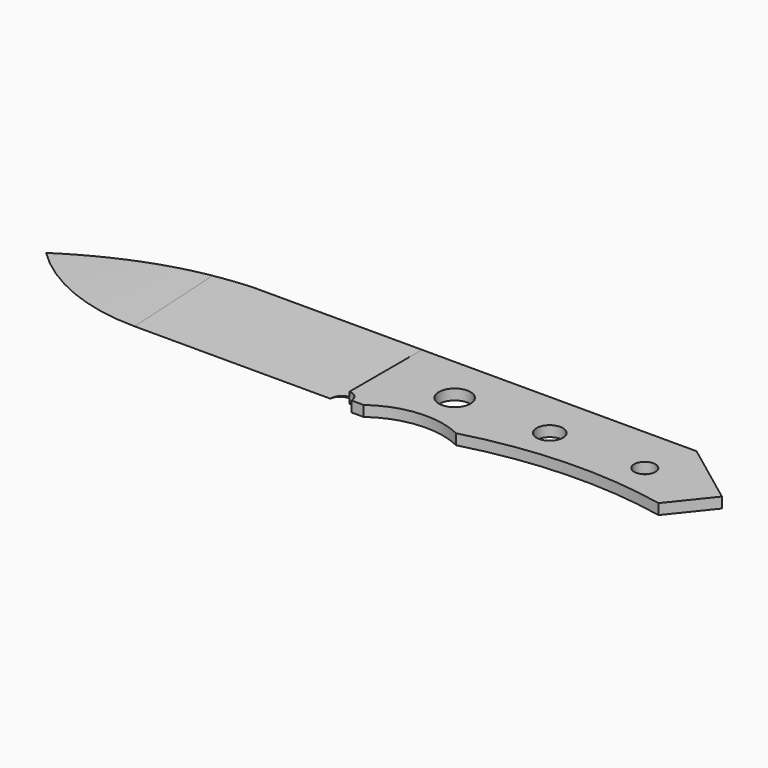
from build123d import *

# Parameters (mm, degrees)
F0_W     = 203.2
F0_H     = 38.1
F1_DEPTH = 3.175
F2_W     = 3.175
F2_H     = 4.445
F3_DEPTH = 25.4


# Not quite as in the source:
# - a feature names something its author has since deleted; it is built from what else it names


with BuildPart() as f1:
    # F0 (on Top) → F1 (new body)
    with BuildSketch(Plane.XY):
        with Locations((101.6, -19.05)):
            Rectangle(F0_W, F0_H)
    extrude(amount=F1_DEPTH)

    # F2 (on face) → F3 (cut)
    with BuildSketch(Plane.XY.offset(3.175)):
        with BuildLine():
            Line((0, -9.525), (0, -14.2875))
            ThreePointArc((0, -14.2875), (24.649723028, -4.4760985439), (50.8, 0))
            Line((50.8, 0), (0, 0))
            Line((0, 0), (0, -9.525))
        make_face()
        with Locations((103.1875, -35.8775)):
            Rectangle(F2_W, F2_H)
        with BuildLine():
            ThreePointArc((104.775, -30.48), (103.8450640303, -32.7250640303), (101.6, -33.655))
            Line((101.6, -33.655), (104.775, -33.655))
            Line((104.775, -33.655), (104.775, -30.48))
        make_face()
        with BuildLine():
            Line((104.775, -30.48), (101.6, -30.48))
            Line((101.6, -30.48), (101.6, -33.655))
            ThreePointArc((101.6, -33.655), (103.8450640303, -32.7250640303), (104.775, -30.48))
        make_face()
        with BuildLine():
            Line((101.6, -27.305), (101.6, -30.48))
            Line((101.6, -30.48), (104.775, -30.48))
            ThreePointArc((104.775, -30.48), (103.8450640303, -28.2349359697), (101.6, -27.305))
        make_face()
        with BuildLine():
            Line((98.4250000029, -30.4801362911), (101.6, -30.48))
            Line((101.6, -30.48), (101.6, -27.305))
            ThreePointArc((101.6, -27.305), (99.3548877841, -28.2349841564), (98.4250000029, -30.4801362911))
        make_face()
        with BuildLine():
            Line((101.6, -33.655), (101.6, -30.48))
            Line((101.6, -30.48), (98.4250000029, -30.4801362911))
            ThreePointArc((98.4250000029, -30.4801362911), (99.3549841564, -32.7251122159), (101.6, -33.655))
        make_face()
        with BuildLine():
            ThreePointArc((108.3690122037, -30.48), (106.4969075417, -31.9824905065), (104.775, -33.655))
            Line((104.775, -33.655), (104.775, -38.1))
            Line((104.775, -38.1), (184.15, -38.1))
            Line((184.15, -38.1), (193.675, -26.19375))
            ThreePointArc((193.675, -26.19375), (163.9135585822, -23.6655567526), (134.3847364187, -28.1581971794))
            ThreePointArc((134.3847364187, -28.1581971794), (121.0555708247, -25.7189035938), (108.3690122037, -30.48))
        make_face()
        with BuildLine():
            Line((101.6, -38.1), (101.6, -33.655))
            ThreePointArc((101.6, -33.655), (99.3549841564, -32.7251122159), (98.4250000029, -30.4801362911))
            Line((98.4250000029, -30.4801362911), (39.6036359929, -30.4826612755))
            ThreePointArc((39.6036359929, -30.4826612755), (18.2099329026, -26.2778753266), (0, -14.2875))
            Line((0, -14.2875), (0, -19.05))
            Line((0, -19.05), (0, -38.1))
            Line((0, -38.1), (101.6, -38.1))
        make_face()
        Polygon((203.2, 0), (184.15, 0), (203.2, -14.2875), align=None)
        Polygon((193.675, -26.19375), (184.15, -38.1), (203.2, -38.1), (203.2, -19.05), (203.2, -14.2875), align=None)
        with BuildLine():
            Line((108.3690122037, -30.48), (104.775, -30.48))
            Line((104.775, -30.48), (104.775, -33.655))
            ThreePointArc((104.775, -33.655), (106.4969075417, -31.9824905065), (108.3690122037, -30.48))
        make_face()
        with BuildLine():
            ThreePointArc((127.6218066335, -14.2875), (122.8593066335, -9.525), (118.0968066335, -14.2875))
            Line((118.0968066335, -14.2875), (127.6218066335, -14.2875))
        make_face()
        with BuildLine():
            Line((127.6218066335, -14.2875), (118.0968066335, -14.2875))
            ThreePointArc((118.0968066335, -14.2875), (122.8593066335, -19.05), (127.6218066335, -14.2875))
        make_face()
        with BuildLine():
            Line((176.8343066335, -14.2875), (183.1843066335, -14.2875))
            ThreePointArc((183.1843066335, -14.2875), (180.0093066335, -11.1125), (176.8343066335, -14.2875))
        make_face()
        with BuildLine():
            ThreePointArc((176.8343066335, -14.2875), (180.0093066335, -17.4625), (183.1843066335, -14.2875))
            Line((183.1843066335, -14.2875), (176.8343066335, -14.2875))
        make_face()
        with BuildLine():
            ThreePointArc((155.4030566335, -14.2875), (151.4343066335, -10.31875), (147.4655566335, -14.2875))
            Line((147.4655566335, -14.2875), (155.4030566335, -14.2875))
        make_face()
        with BuildLine():
            Line((155.4030566335, -14.2875), (147.4655566335, -14.2875))
            ThreePointArc((147.4655566335, -14.2875), (151.4343066335, -18.25625), (155.4030566335, -14.2875))
        make_face()
    extrude(amount=-F3_DEPTH, mode=Mode.SUBTRACT)

    # F8: sweep along a path in F5
    with BuildLine(Plane.XY.offset(1.5875)) as f8_path:
        Line((101.6, -30.48), (39.6036359929, -30.4826612755))
        ThreePointArc((39.6036359929, -30.4826612755), (18.2099329026, -26.2778753266), (0, -14.2875))
    # F7 (on offset) → F8 (sweep, cut)
    with BuildSketch(Plane.YZ.offset(101.6)):
        Polygon((-30.48, 3.1877), (-30.48, 1.5875), (-21.4048148322, 3.1877), align=None)
        Polygon((-21.4048148322, 3.1877), (-30.48, 1.5875), (0, 3.1877), align=None)
        Polygon((-21.4768401114, 0), (0, 0), (-30.48, 1.5875), align=None)
        Polygon((-4.1187478461, -3.0607), (-21.4768401114, 0), (-30.48, 0), (-30.48, -3.0607), align=None)
        Polygon((-30.48, 0), (-21.4768401114, 0), (-30.48, 1.5875), align=None)
        Polygon((-30.48, 6.2357), (-30.48, 3.1877), (-21.4048148322, 3.1877), (-4.1187478461, 6.2357), align=None)
    sweep(path=f8_path.line, mode=Mode.SUBTRACT)


solid = f1.part
